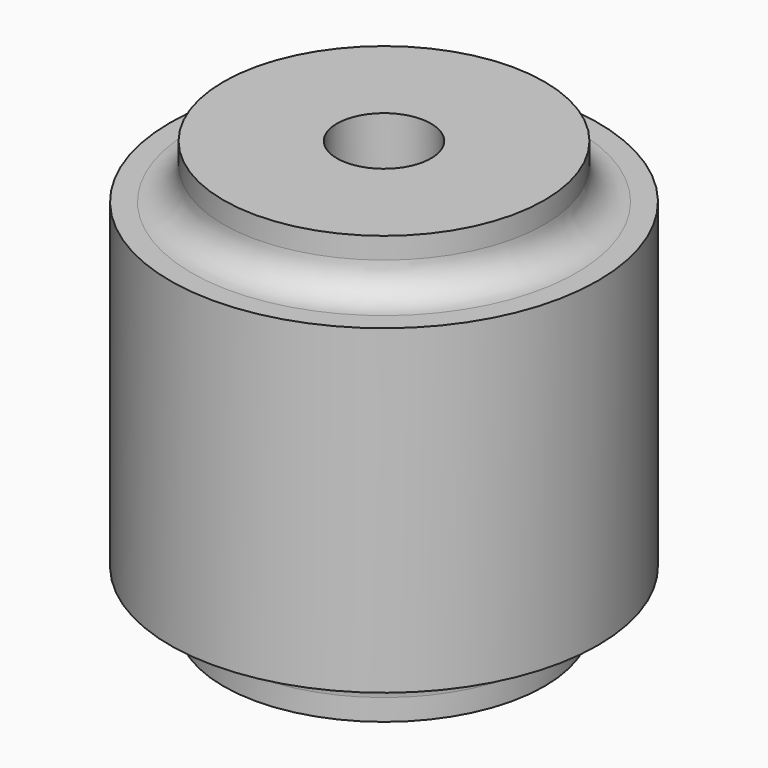
from build123d import *

# Parameters (mm, degrees)
F2_R           = 3
F5_D           = 8.8
F5_DEPTH       = 10
F5_TIP         = 2.6437867237
F5_ON_F3_D     = 8.8
F5_ON_F3_DEPTH = 10
F5_ON_F3_TIP   = 2.6437867237


with BuildPart() as f1:
    # F0 (on Front) → F1 (revolve)
    with BuildSketch(Plane.XZ):
        Polygon((0, -20), (0, 20), (-15, 20), (-15, 15), (-20, 15), (-20, -15), (-15, -15), (-15, -20), align=None)
    revolve(axis=Axis((0, 0, 0), (0, 0, -1)))

    # F2
    f2_edges = [f1.edges().sort_by_distance(p)[0] for p in [
        (15, 0, 15),
        (15, 0, -15),
    ]]
    fillet(f2_edges, radius=F2_R)

    # F5
    with Locations(Plane(origin=(0, 0, -20), x_dir=(1, 0, 0), z_dir=(0, 0, -1))):
        with Locations((0, 0)):
            Hole(F5_D / 2, depth=F5_DEPTH)
            with Locations((0, 0, -(F5_DEPTH + F5_TIP / 2))):  # 118° drill point
                Cone(0, F5_D / 2, F5_TIP, mode=Mode.SUBTRACT)

    # F5 on F3
    with Locations(Plane.XY.offset(20)):
        with Locations((0, 0)):
            Hole(F5_ON_F3_D / 2, depth=F5_ON_F3_DEPTH)
            with Locations((0, 0, -(F5_ON_F3_DEPTH + F5_ON_F3_TIP / 2))):  # 118° drill point
                Cone(0, F5_ON_F3_D / 2, F5_ON_F3_TIP, mode=Mode.SUBTRACT)


solid = f1.part
